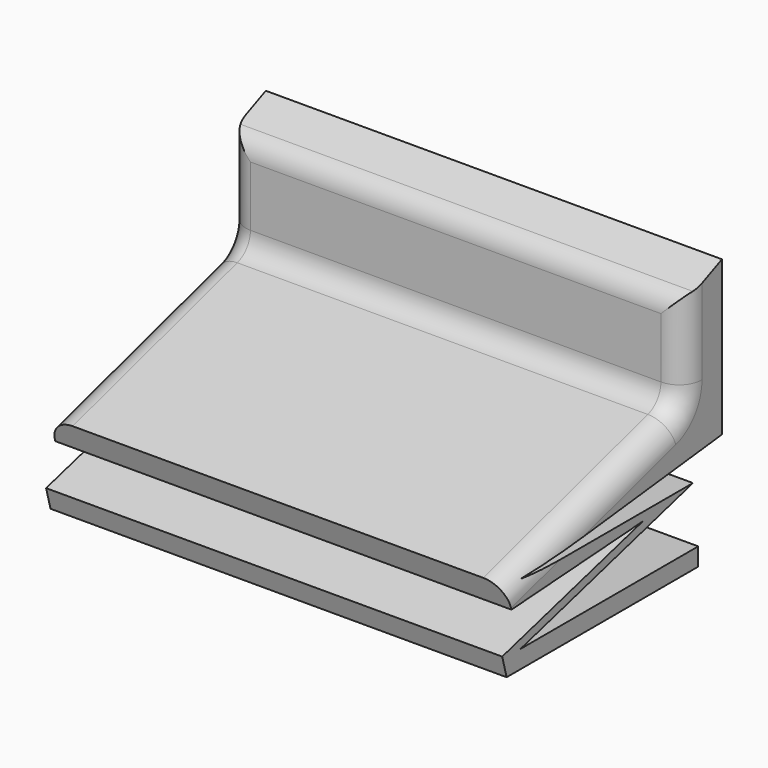
from build123d import *

# Parameters (mm, degrees)
F1_DEPTH     = 101.6
F2_T1_DEPTH  = 101.6
F2_T3_DEPTH  = 118.1792407144
F2_T5_DEPTH  = 29.422869264
F2_T7_DEPTH  = 60.4590704492
F2_T10_ANGLE = 73.6909129446
F2_T12_ANGLE = 73.6909129446


# Not quite as in the source:
# - a fillet or chamfer that OpenCascade refuses, or shapes differently, is made with other operations: its cross-section is extruded or revolved along the edge and cut away or added


with BuildPart() as f1:
    # F0 (on Right) → F1 (new body)
    with BuildSketch(Plane.YZ):
        Polygon((15.3971137479, -57.599131723), (15.3971137479, -53.6149479449), (-34.0936109424, -53.6149479449), (13.9307221398, -40.600720793), (-33.1771150231, -40.600720793), (21.9958759844, -34.3685559928), (21.9958759844, 0), (11.3645363599, -4.6741236001), (11.3645363599, -25.2036079764), (-38.1261855364, -39.6842285991), (-36.6007449852, -44.8977588791), (0, -42.4337126315), (-39.1800553827, -53.0512081353), (-37.9476028562, -57.599131723), align=None)
    extrude(amount=F1_DEPTH)

    # F2: fillet of radius 5.08 on 6 edges, made by hand

    # F2_s2 → F2_t1 (join)
    with BuildSketch(Plane.YZ):
        with BuildLine():
            ThreePointArc((11.3645363599, -21.3969928641), (10.3498362027, -24.44325897), (7.7110965222, -26.2725775576))
            Line((7.7110965222, -26.2725775576), (11.3645363599, -25.2036079764))
            Line((11.3645363599, -25.2036079764), (11.3645363599, -21.3969928641))
        make_face()
    extrude(amount=F2_T1_DEPTH)

    # F2_s4 → F2_t3 (cut)
    with BuildSketch(Plane.YZ.offset(-8.2896203572)):
        with BuildLine():
            ThreePointArc((14.3999677165, -3.3395804625), (12.1905494824, -5.2132838517), (11.3645363599, -7.989971743))
            Line((11.3645363599, -7.989971743), (11.3645363599, -4.6741236001))
            Line((11.3645363599, -4.6741236001), (14.3999677165, -3.3395804625))
        make_face()
    extrude(amount=F2_T3_DEPTH, mode=Mode.SUBTRACT)

    # F2_s6 → F2_t5 (cut)
    with BuildSketch(Plane.XY.offset(-21.3969928641)):
        with BuildLine():
            ThreePointArc((0, 16.4445363599), (1.4878975516, 12.8524339115), (5.08, 11.3645363599))
            Line((5.08, 11.3645363599), (0, 11.3645363599))
            Line((0, 11.3645363599), (0, 16.4445363599))
        make_face()
        with BuildLine():
            ThreePointArc((101.6, 16.4445363599), (100.1121024484, 12.8524339115), (96.52, 11.3645363599))
            Line((96.52, 11.3645363599), (101.6, 11.3645363599))
            Line((101.6, 11.3645363599), (101.6, 16.4445363599))
        make_face()
    extrude(amount=F2_T5_DEPTH, mode=Mode.SUBTRACT)

    # F2_s8 → F2_t7 (cut)
    with BuildSketch(Plane(origin=(0, 0.0220464736, 0.0064506358), x_dir=(1, 0, 0), z_dir=(0, -0.9597607664, -0.2808189296))):
        with BuildLine():
            ThreePointArc((0, -32.4608110442), (1.4878975516, -28.8687085958), (5.08, -27.3808110442))
            Line((5.08, -27.3808110442), (0, -27.3808110442))
            Line((0, -27.3808110442), (0, -32.4608110442))
        make_face()
        with BuildLine():
            ThreePointArc((101.6, -32.4608110442), (100.1121024484, -28.8687085958), (96.52, -27.3808110442))
            Line((96.52, -27.3808110442), (101.6, -27.3808110442))
            Line((101.6, -27.3808110442), (101.6, -32.4608110442))
        make_face()
    extrude(amount=F2_T7_DEPTH, mode=Mode.SUBTRACT)

    # F2_s9 → F2_t10 (revolve, cut)
    with BuildSketch(Plane.XY.offset(-21.3969928641)):
        with BuildLine():
            ThreePointArc((101.6, 16.4445363599), (100.1121024484, 12.8524339115), (96.52, 11.3645363599))
            Line((96.52, 11.3645363599), (101.6, 11.3645363599))
            Line((101.6, 11.3645363599), (101.6, 16.4445363599))
        make_face()
    revolve(axis=Axis((101.6, 6.2845363599, -21.3969928641), (-1, 0, 0)), revolution_arc=F2_T10_ANGLE, mode=Mode.SUBTRACT)

    # F2_s11 → F2_t12 (revolve, cut)
    with BuildSketch(Plane.XY.offset(-21.3969928641)):
        with BuildLine():
            ThreePointArc((0, 16.4445363599), (1.4878975516, 12.8524339115), (5.08, 11.3645363599))
            Line((5.08, 11.3645363599), (0, 11.3645363599))
            Line((0, 11.3645363599), (0, 16.4445363599))
        make_face()
    revolve(axis=Axis((0, 6.2845363599, -21.3969928641), (-1, 0, 0)), revolution_arc=F2_T12_ANGLE, mode=Mode.SUBTRACT)


solid = f1.part
